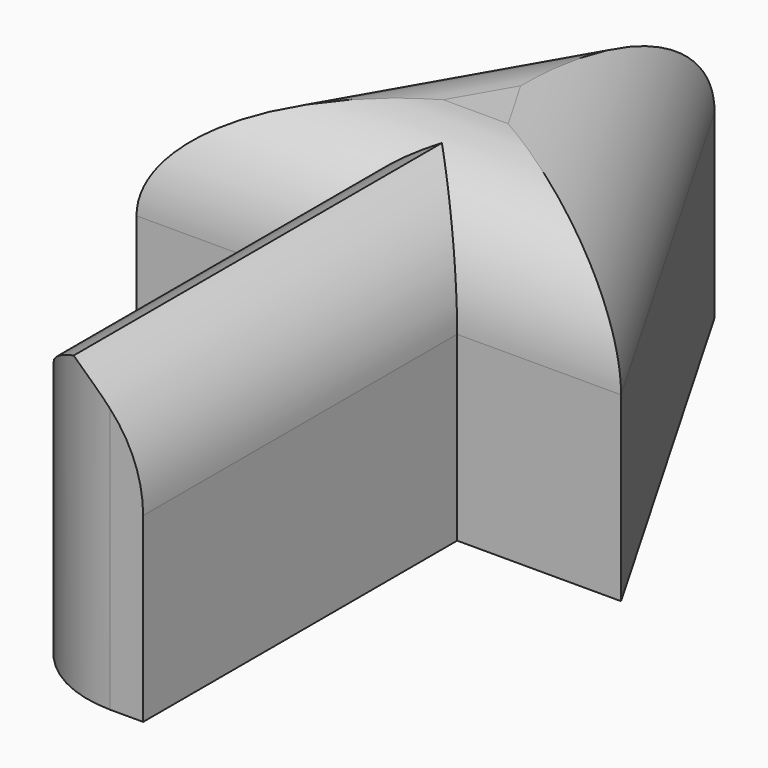
from build123d import *

# Parameters (mm, degrees)
F1_DEPTH     = 12.7
F2_W         = 6.4008012414
F2_H         = 16.7640000582
F3_DEPTH     = 12.7
F4_T1_DEPTH  = 19.5733811916
F4_T3_DEPTH  = 19.745817567
F4_T5_DEPTH  = 29.1591995999
F4_T10_DEPTH = 32.2733811916
F4_T15_DEPTH = 32.445817567
F4_T21_DEPTH = 32.2733811916
F4_T26_DEPTH = 41.8591995999
F4_T33_DEPTH = 32.445817567
F4_T38_DEPTH = 41.8591995999
F5_T1_DEPTH  = 39.8541212651
F5_T3_DEPTH  = 39.8541212651
F6_T1_DEPTH  = 33.0248285058


# Not quite as in the source:
# - a fillet or chamfer that OpenCascade refuses, or shapes differently, is made with other operations: its cross-section is extruded or revolved along the edge and cut away or added


with BuildPart() as f1:
    # F0 (on Top) → F1 (new body)
    with BuildSketch(Plane.XY):
        Polygon((-38.5418191015, 11.7347994819), (-48.7018191015, 29.3324356868), (-58.8618191015, 11.7347994819), align=None)
    extrude(amount=F1_DEPTH)

    # F2 (on Top) → F3 (join)
    with BuildSketch(Plane.XY):
        with Locations((-48.6156009138, 3.6575999111)):
            Rectangle(F2_W, F2_H)
    extrude(amount=F3_DEPTH)

    # F4: fillet of radius 5.08 on 4 edges, made by hand

    # F4_s2 → F4_t1 (cut)
    with BuildSketch(Plane.YZ.offset(-45.4152002931)):
        with BuildLine():
            ThreePointArc((11.7347994819, 7.62), (13.2226970335, 11.2121024484), (16.8147994819, 12.7))
            Line((16.8147994819, 12.7), (11.7347994819, 12.7))
            Line((11.7347994819, 12.7), (11.7347994819, 7.62))
        make_face()
    extrude(amount=F4_T1_DEPTH, mode=Mode.SUBTRACT)

    # F4_s4 → F4_t3 (cut)
    with BuildSketch(Plane.YZ.offset(-71.5618191015)):
        with BuildLine():
            ThreePointArc((16.8147994819, 12.7), (13.2226970335, 11.2121024484), (11.7347994819, 7.62))
            Line((11.7347994819, 7.62), (11.7347994819, 12.7))
            Line((11.7347994819, 12.7), (16.8147994819, 12.7))
        make_face()
    extrude(amount=F4_T3_DEPTH, mode=Mode.SUBTRACT)

    # F4_s6 → F4_t5 (cut)
    with BuildSketch(Plane.XZ.offset(-11.7347994819)):
        with BuildLine():
            ThreePointArc((-50.4952002931, 12.7), (-46.9030978446, 11.2121024484), (-45.4152002931, 7.62))
            Line((-45.4152002931, 7.62), (-45.4152002931, 12.7))
            Line((-45.4152002931, 12.7), (-50.4952002931, 12.7))
        make_face()
        with BuildLine():
            ThreePointArc((-46.7360015345, 12.7), (-50.3281039829, 11.2121024484), (-51.8160015345, 7.62))
            Line((-51.8160015345, 7.62), (-51.8160015345, 12.7))
            Line((-51.8160015345, 12.7), (-46.7360015345, 12.7))
        make_face()
    extrude(amount=F4_T5_DEPTH, mode=Mode.SUBTRACT)


with BuildPart() as f4_tool8:
    # F4_s9 → F4_t10 (new body)
    with BuildSketch(Plane.YZ.offset(-58.1152002931)):
        with BuildLine():
            ThreePointArc((11.7347994819, 7.62), (13.2226970335, 11.2121024484), (16.8147994819, 12.7))
            Line((16.8147994819, 12.7), (11.7347994819, 12.7))
            Line((11.7347994819, 12.7), (11.7347994819, 7.62))
        make_face()
    extrude(amount=F4_T10_DEPTH)

    split(bisect_by=Plane.YZ.offset(-51.8160015345), keep=Keep.BOTTOM)


with BuildPart() as f1_1:
    add(f1.part)

    # F4_t7: cut F4_tool8
    add(f4_tool8.part, mode=Mode.SUBTRACT)


with BuildPart() as f4_tool13:
    # F4_s14 → F4_t15 (new body)
    with BuildSketch(Plane.YZ.offset(-71.5618191015)):
        with BuildLine():
            ThreePointArc((16.8147994819, 12.7), (13.2226970335, 11.2121024484), (11.7347994819, 7.62))
            Line((11.7347994819, 7.62), (11.7347994819, 12.7))
            Line((11.7347994819, 12.7), (16.8147994819, 12.7))
        make_face()
    extrude(amount=F4_T15_DEPTH)

    split(bisect_by=Plane.YZ.offset(-45.4152002931), keep=Keep.TOP)


with BuildPart() as f1_2:
    add(f1_1.part)

    # F4_t12: cut F4_tool13
    add(f4_tool13.part, mode=Mode.SUBTRACT)


with BuildPart() as f4_tool19:
    # F4_s20 → F4_t21 (new body)
    with BuildSketch(Plane.YZ.offset(-58.1152002931)):
        with BuildLine():
            ThreePointArc((11.7347994819, 7.62), (13.2226970335, 11.2121024484), (16.8147994819, 12.7))
            Line((16.8147994819, 12.7), (11.7347994819, 12.7))
            Line((11.7347994819, 12.7), (11.7347994819, 7.62))
        make_face()
    extrude(amount=F4_T21_DEPTH)

    split(bisect_by=Plane.YZ.offset(-45.4152002931), keep=Keep.BOTTOM)

    split(bisect_by=Plane.YZ.offset(-51.8160015345), keep=Keep.TOP)


with BuildPart() as f4_tool24:
    # F4_s25 → F4_t26 (new body)
    with BuildSketch(Plane.XZ.offset(17.424400118)):
        with BuildLine():
            ThreePointArc((-50.4952002931, 12.7), (-46.9030978446, 11.2121024484), (-45.4152002931, 7.62))
            Line((-45.4152002931, 7.62), (-45.4152002931, 12.7))
            Line((-45.4152002931, 12.7), (-50.4952002931, 12.7))
        make_face()
    extrude(amount=-F4_T26_DEPTH)

    split(bisect_by=Plane.XZ.offset(-11.7347994819), keep=Keep.BOTTOM)


with BuildPart() as f4_tool19_1:
    add(f4_tool19.part)

    # F4_t28: intersect F4_tool24
    add(f4_tool24.part, mode=Mode.INTERSECT)


with BuildPart() as f1_3:
    add(f1_2.part)

    # F4_t17: cut F4_tool19
    add(f4_tool19_1.part, mode=Mode.SUBTRACT)


with BuildPart() as f4_tool31:
    # F4_s32 → F4_t33 (new body)
    with BuildSketch(Plane.YZ.offset(-71.5618191015)):
        with BuildLine():
            ThreePointArc((16.8147994819, 12.7), (13.2226970335, 11.2121024484), (11.7347994819, 7.62))
            Line((11.7347994819, 7.62), (11.7347994819, 12.7))
            Line((11.7347994819, 12.7), (16.8147994819, 12.7))
        make_face()
    extrude(amount=F4_T33_DEPTH)

    split(bisect_by=Plane.YZ.offset(-45.4152002931), keep=Keep.BOTTOM)

    split(bisect_by=Plane.YZ.offset(-51.8160015345), keep=Keep.TOP)


with BuildPart() as f4_tool36:
    # F4_s37 → F4_t38 (new body)
    with BuildSketch(Plane.XZ.offset(-24.4347994819)):
        with BuildLine():
            ThreePointArc((-46.7360015345, 12.7), (-50.3281039829, 11.2121024484), (-51.8160015345, 7.62))
            Line((-51.8160015345, 7.62), (-51.8160015345, 12.7))
            Line((-51.8160015345, 12.7), (-46.7360015345, 12.7))
        make_face()
    extrude(amount=F4_T38_DEPTH)

    split(bisect_by=Plane.XZ.offset(-11.7347994819), keep=Keep.BOTTOM)


with BuildPart() as f4_tool31_1:
    add(f4_tool31.part)

    # F4_t40: intersect F4_tool36
    add(f4_tool36.part, mode=Mode.INTERSECT)


with BuildPart() as f1_4:
    add(f1_3.part)

    # F4_t29: cut F4_tool31
    add(f4_tool31_1.part, mode=Mode.SUBTRACT)

    # F5: fillet of radius 5.08 on 2 edges, made by hand

    # F5_s2 → F5_t1 (cut)
    with BuildSketch(Plane(origin=(6.8758624545, 11.909343117, 0), x_dir=(0, 0, 1), z_dir=(-0.5, -0.8660254038, 0))):
        with BuildLine():
            ThreePointArc((12.7, 51.7632303958), (11.2121024484, 55.3553328442), (7.62, 56.8432303958))
            Line((7.62, 56.8432303958), (12.7, 56.8432303958))
            Line((12.7, 56.8432303958), (12.7, 51.7632303958))
        make_face()
    extrude(amount=F5_T1_DEPTH, mode=Mode.SUBTRACT)

    # F5_s4 → F5_t3 (cut)
    with BuildSketch(Plane(origin=(-11.2997113727, 19.5716742083, 0), x_dir=(0, 0, 1), z_dir=(-0.5, 0.8660254038, 0))):
        with BuildLine():
            ThreePointArc((7.62, -27.510794709), (11.2121024484, -28.9986922605), (12.7, -32.590794709))
            Line((12.7, -32.590794709), (12.7, -27.510794709))
            Line((12.7, -27.510794709), (7.62, -27.510794709))
        make_face()
    extrude(amount=F5_T3_DEPTH, mode=Mode.SUBTRACT)

    # F6: fillet of radius 5.08 on 2 edges, made by hand

    # F6_s2 → F6_t1 (cut)
    with BuildSketch(Plane.XY.offset(-12.7024142529)):
        with BuildLine():
            ThreePointArc((-51.8164015345, 0.3565655674), (-50.3281039829, -3.2365025664), (-46.735035849, -4.724800118))
            Line((-46.735035849, -4.724800118), (-46.735035849, -5.2329366865))
            ThreePointArc((-46.735035849, -5.2329366865), (-49.2755186917, -5.2325366865), (-51.8160015345, -5.2325366865))
            Line((-51.8160015345, -5.2325366865), (-52.324138103, -4.724400118))
            ThreePointArc((-52.324138103, -4.724400118), (-52.324138103, -2.1839172753), (-52.324538103, 0.3565655674))
            Line((-52.324538103, 0.3565655674), (-51.8164015345, 0.3565655674))
        make_face()
    extrude(amount=F6_T1_DEPTH, mode=Mode.SUBTRACT)


solid = f1_4.part
